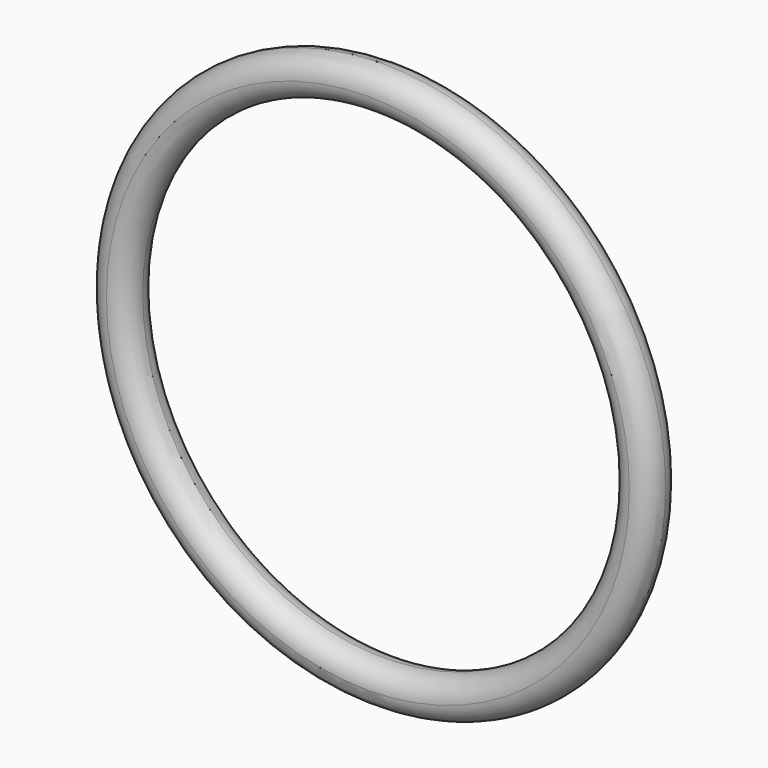
from build123d import *

# Parameters (mm, degrees)
F0_R     = 10.5
F0_R_2   = 9
F1_DEPTH = 1.5
F2_R     = 0.74999


# Not quite as in the source:
# - a fillet or chamfer is up to 0.001 mm smaller than in the source, because OpenCascade refuses the exact size


with BuildPart() as f1:
    # F0 (on Front) → F1 (new body)
    with BuildSketch(Plane.XZ):
        Circle(F0_R)
        Circle(F0_R_2, mode=Mode.SUBTRACT)
    extrude(amount=F1_DEPTH)

    # F2 (radius 0.75 in the source; OpenCascade refuses exactly that, so slightly less here)
    f2_edges = [f1.edges().sort_by_distance(p)[0] for p in [
        (-9, -1.5, 0),
        (-10.5, -1.5, 0),
        (-9, 0, 0),
        (-10.5, 0, 0),
    ]]
    fillet(f2_edges, radius=F2_R)


solid = f1.part
